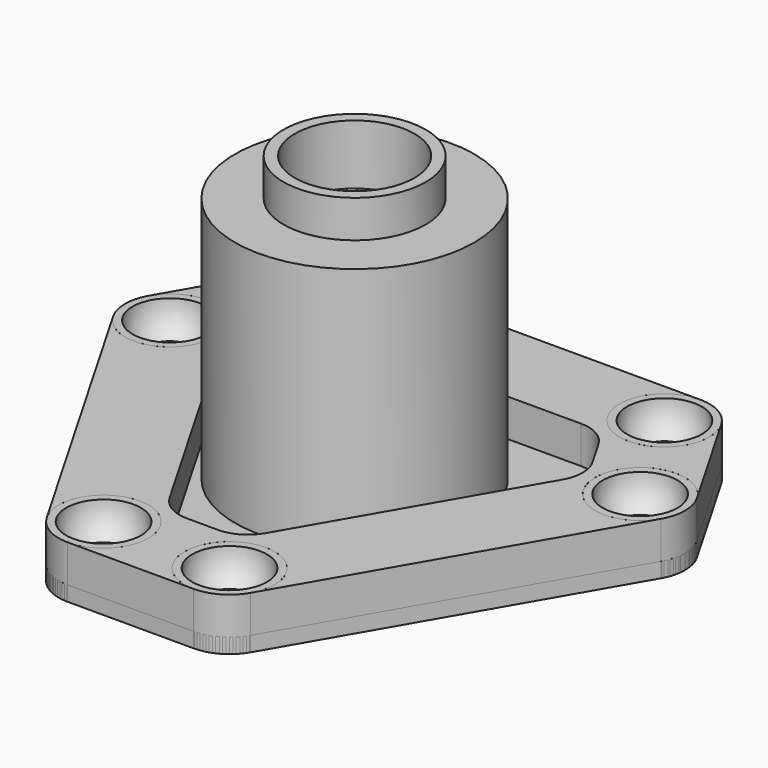
from build123d import *

# Parameters (mm, degrees)
F0_R      = 6
F1_DEPTH  = 7
F2_R      = 5
F3_DEPTH  = 5
F4_R      = 4.99999
F5_R      = 4.25
F6_DEPTH  = 3
F9_COUNT  = 3
F10_R     = 4.25
F11_DEPTH = 2
F13_DEPTH = 5
F14_R     = 13
F15_DEPTH = 2.001
F16_R     = 16
F17_DEPTH = 30
F18_R     = 13
F19_DEPTH = 30.001
F20_R     = 16
F21_DEPTH = 3
F22_R     = 8
F23_DEPTH = 3
F24_R     = 9.5
F24_R_2   = 8
F25_DEPTH = 5
F28_DEPTH = 15


# Not quite as in the source:
# - a fillet or chamfer is up to 0.001 mm smaller than in the source, because OpenCascade refuses the exact size


with BuildPart() as f1:
    # F0 (on Top) → F1 (new body)
    with BuildSketch(Plane.XY):
        with Locations((-23, 23)):
            Circle(F0_R)
    extrude(amount=F1_DEPTH)

    # F2 (on face) → F3 (cut)
    with BuildSketch(Plane.XY.offset(7)):
        with Locations((-23, 23)):
            Circle(F2_R)
    extrude(amount=-F3_DEPTH, mode=Mode.SUBTRACT)

    # F4 (radius 5 in the source; OpenCascade refuses exactly that, so slightly less here)
    f4_edges = [f1.edges().sort_by_distance(p)[0] for p in [
        (-28, 23, 2),
    ]]
    fillet(f4_edges, radius=F4_R)

    # F5 (on face) → F6 (cut)
    with BuildSketch(Plane(origin=(0, 0, 0), x_dir=(1, 0, 0), z_dir=(0, 0, -1))):
        with Locations((-23, -23)):
            Circle(F5_R)
    extrude(amount=-F6_DEPTH, mode=Mode.SUBTRACT)


with BuildPart() as f7_1:
    # F7: instance of F1
    add(f1.part.mirror(Plane.YZ))


with BuildPart() as f9_1:
    # F9: instance of F1
    add(f1.part.rotate(Axis((0, 0, 26.5737418085), (0, 0, 1)), 1 * 360 / F9_COUNT))


with BuildPart() as f9_2:
    # F9: instance of F1
    add(f1.part.rotate(Axis((0, 0, 26.5737418085), (0, 0, 1)), 2 * 360 / F9_COUNT))


with BuildPart() as f9_3:
    # F9: instance of F7_1
    add(f7_1.part.rotate(Axis((0, 0, 26.5737418085), (0, 0, 1)), 1 * 360 / F9_COUNT))


with BuildPart() as f9_4:
    # F9: instance of F7_1
    add(f7_1.part.rotate(Axis((0, 0, 26.5737418085), (0, 0, 1)), 2 * 360 / F9_COUNT))


with BuildPart() as f11:
    # F10 (on Top) → F11 (new body)
    with BuildSketch(Plane.XY):
        with BuildLine():
            ThreePointArc((29, 23), (18.7573593129, 18.7573593129), (23, 29))
            Line((23, 29), (-23, 29))
            ThreePointArc((-23, 29), (-18.7573593129, 27.2426406871), (-17, 23))
            ThreePointArc((-17, 23), (-24.5529142706, 17.2044450423), (-28.1961524227, 26))
            Line((-28.1961524227, 26), (-36.6147367097, 11.418584287))
            ThreePointArc((-36.6147367097, 11.418584287), (-29.8656700164, 14.2141392448), (-25.418584287, 8.418584287))
            ThreePointArc((-25.418584287, 8.418584287), (-29.8656700164, 2.6230293293), (-36.6147367097, 5.418584287))
            Line((-36.6147367097, 5.418584287), (-13.6147367097, -34.418584287))
            ThreePointArc((-13.6147367097, -34.418584287), (-9.9714985577, -25.6230293293), (-2.418584287, -31.418584287))
            ThreePointArc((-2.418584287, -31.418584287), (-4.1759435999, -35.6612249742), (-8.418584287, -37.418584287))
            Line((-8.418584287, -37.418584287), (8.418584287, -37.418584287))
            ThreePointArc((8.418584287, -37.418584287), (4.1759435999, -27.1759435999), (14.418584287, -31.418584287))
            ThreePointArc((14.418584287, -31.418584287), (14.2141392448, -32.9714985577), (13.6147367097, -34.418584287))
            Line((13.6147367097, -34.418584287), (36.6147367097, 5.418584287))
            ThreePointArc((36.6147367097, 5.418584287), (25.418584287, 8.418584287), (36.6147367097, 11.418584287))
            Line((36.6147367097, 11.418584287), (28.1961524227, 26))
            ThreePointArc((28.1961524227, 26), (28.7955549577, 24.5529142706), (29, 23))
        make_face()
        with BuildLine():
            ThreePointArc((28.1961524227, 26), (26, 28.1961524227), (23, 29))
            ThreePointArc((23, 29), (18.7573593129, 18.7573593129), (29, 23))
            ThreePointArc((29, 23), (28.7955549577, 24.5529142706), (28.1961524227, 26))
        make_face()
        with Locations((23, 23)):
            Circle(F10_R, mode=Mode.SUBTRACT)
        with BuildLine():
            ThreePointArc((-17, 23), (-18.7573593129, 27.2426406871), (-23, 29))
            ThreePointArc((-23, 29), (-26, 28.1961524227), (-28.1961524227, 26))
            ThreePointArc((-28.1961524227, 26), (-24.5529142706, 17.2044450423), (-17, 23))
        make_face()
        with Locations((-23, 23)):
            Circle(F10_R, mode=Mode.SUBTRACT)
        with BuildLine():
            ThreePointArc((37.418584287, 8.418584287), (37.2141392448, 9.9714985577), (36.6147367097, 11.418584287))
            ThreePointArc((36.6147367097, 11.418584287), (25.418584287, 8.418584287), (36.6147367097, 5.418584287))
            ThreePointArc((36.6147367097, 5.418584287), (37.2141392448, 6.8656700164), (37.418584287, 8.418584287))
        make_face()
        with Locations((31.418584287, 8.418584287)):
            Circle(F10_R, mode=Mode.SUBTRACT)
        with BuildLine():
            ThreePointArc((-25.418584287, 8.418584287), (-29.8656700164, 14.2141392448), (-36.6147367097, 11.418584287))
            ThreePointArc((-36.6147367097, 11.418584287), (-37.418584287, 8.418584287), (-36.6147367097, 5.418584287))
            ThreePointArc((-36.6147367097, 5.418584287), (-29.8656700164, 2.6230293293), (-25.418584287, 8.418584287))
        make_face()
        with Locations((-31.418584287, 8.418584287)):
            Circle(F10_R, mode=Mode.SUBTRACT)
        with BuildLine():
            ThreePointArc((8.418584287, -37.418584287), (11.418584287, -36.6147367097), (13.6147367097, -34.418584287))
            ThreePointArc((13.6147367097, -34.418584287), (14.2141392448, -32.9714985577), (14.418584287, -31.418584287))
            ThreePointArc((14.418584287, -31.418584287), (4.1759435999, -27.1759435999), (8.418584287, -37.418584287))
        make_face()
        with Locations((8.418584287, -31.418584287)):
            Circle(F10_R, mode=Mode.SUBTRACT)
        with BuildLine():
            ThreePointArc((-2.418584287, -31.418584287), (-9.9714985577, -25.6230293293), (-13.6147367097, -34.418584287))
            ThreePointArc((-13.6147367097, -34.418584287), (-11.418584287, -36.6147367097), (-8.418584287, -37.418584287))
            ThreePointArc((-8.418584287, -37.418584287), (-4.1759435999, -35.6612249742), (-2.418584287, -31.418584287))
        make_face()
        with Locations((-8.418584287, -31.418584287)):
            Circle(F10_R, mode=Mode.SUBTRACT)
    extrude(amount=F11_DEPTH)

    # F14 (on face) → F15 (cut, through all)
    with BuildSketch(Plane.XY.offset(2)):
        Circle(F14_R)
    extrude(amount=-F15_DEPTH, mode=Mode.SUBTRACT)

    # F16 (on face) → F17 (join)
    with BuildSketch(Plane.XY.offset(2)):
        Circle(F16_R)
    extrude(amount=F17_DEPTH)

    # F18 (on face) → F19 (cut, through all)
    with BuildSketch(Plane(origin=(0, 0, 2), x_dir=(1, 0, 0), z_dir=(0, 0, -1))):
        Circle(F18_R)
    extrude(amount=-F19_DEPTH, mode=Mode.SUBTRACT)

    # F20 (on face) → F21 (join)
    with BuildSketch(Plane.XY.offset(32)):
        Circle(F20_R)
    extrude(amount=F21_DEPTH)

    # F22 (on face) → F23 (cut)
    with BuildSketch(Plane.XY.offset(35)):
        Circle(F22_R)
    extrude(amount=-F23_DEPTH, mode=Mode.SUBTRACT)

    # F24 (on face) → F25 (join)
    with BuildSketch(Plane.XY.offset(35)):
        Circle(F24_R)
        Circle(F24_R_2, mode=Mode.SUBTRACT)
    extrude(amount=F25_DEPTH)

    # F27 (on offset) → F28 (cut)
    with BuildSketch(Plane(origin=(-15.0849364905, 8.7092921435, 0), x_dir=(0.5, 0.8660254038, 0), z_dir=(0.8660254038, -0.5, 0))):
        with BuildLine():
            Line((-1, 30), (-1, 8))
            ThreePointArc((-1, 8), (0, 7), (1, 8))
            Line((1, 8), (1, 30))
            ThreePointArc((1, 30), (0, 31), (-1, 30))
        make_face()
        with BuildLine():
            Line((4, 30), (4, 8))
            ThreePointArc((4, 8), (5, 7), (6, 8))
            Line((6, 8), (6, 30))
            ThreePointArc((6, 30), (5, 31), (4, 30))
        make_face()
        with BuildLine():
            Line((9, 30), (9, 8))
            ThreePointArc((9, 8), (10, 7), (11, 8))
            Line((11, 8), (11, 30))
            ThreePointArc((11, 30), (10, 31), (9, 30))
        make_face()
        with BuildLine():
            Line((-5.9996371421, 30.0602365921), (-5.9996371421, 8.0602365921))
            ThreePointArc((-5.9996371421, 8.0602365921), (-4.9996371421, 7.0602365921), (-3.9996371421, 8.0602365921))
            Line((-3.9996371421, 8.0602365921), (-3.9996371421, 30.0602365921))
            ThreePointArc((-3.9996371421, 30.0602365921), (-4.9996371421, 31.0602365921), (-5.9996371421, 30.0602365921))
        make_face()
        with BuildLine():
            Line((-10.9992742843, 30.1204731841), (-10.9992742843, 8.1204731841))
            ThreePointArc((-10.9992742843, 8.1204731841), (-9.9992742843, 7.1204731841), (-8.9992742843, 8.1204731841))
            Line((-8.9992742843, 8.1204731841), (-8.9992742843, 30.1204731841))
            ThreePointArc((-8.9992742843, 30.1204731841), (-9.9992742843, 31.1204731841), (-10.9992742843, 30.1204731841))
        make_face()
    extrude(amount=F28_DEPTH, mode=Mode.SUBTRACT)


with BuildPart() as f13:
    # F12 (on face) → F13 (new body)
    with BuildSketch(Plane.XY.offset(2)):
        with BuildLine():
            ThreePointArc((28.1961524227, 26), (28.7955549577, 24.5529142706), (29, 23))
            ThreePointArc((29, 23), (18.7573593129, 18.7573593129), (23, 29))
            Line((23, 29), (-23, 29))
            ThreePointArc((-23, 29), (-18.7573593129, 27.2426406871), (-17, 23))
            ThreePointArc((-17, 23), (-24.5529142706, 17.2044450423), (-28.1961524227, 26))
            Line((-28.1961524227, 26), (-36.6147367097, 11.418584287))
            ThreePointArc((-36.6147367097, 11.418584287), (-29.8656700164, 14.2141392448), (-25.418584287, 8.418584287))
            ThreePointArc((-25.418584287, 8.418584287), (-29.8656700164, 2.6230293293), (-36.6147367097, 5.418584287))
            Line((-36.6147367097, 5.418584287), (-13.6147367097, -34.418584287))
            ThreePointArc((-13.6147367097, -34.418584287), (-9.9714985577, -25.6230293293), (-2.418584287, -31.418584287))
            ThreePointArc((-2.418584287, -31.418584287), (-4.1759435999, -35.6612249742), (-8.418584287, -37.418584287))
            Line((-8.418584287, -37.418584287), (8.418584287, -37.418584287))
            ThreePointArc((8.418584287, -37.418584287), (4.1759435999, -27.1759435999), (14.418584287, -31.418584287))
            ThreePointArc((14.418584287, -31.418584287), (14.2141392448, -32.9714985577), (13.6147367097, -34.418584287))
            Line((13.6147367097, -34.418584287), (36.6147367097, 5.418584287))
            ThreePointArc((36.6147367097, 5.418584287), (25.418584287, 8.418584287), (36.6147367097, 11.418584287))
            Line((36.6147367097, 11.418584287), (28.1961524227, 26))
        make_face()
        with BuildLine():
            Line((-16.6491470389, 17), (16.6491470389, 17))
            ThreePointArc((16.6491470389, 17), (19.1491470389, 16.3301270189), (20.9792740578, 14.5))
            Line((20.9792740578, 14.5), (23.0470053838, 10.918584287))
            ThreePointArc((23.0470053838, 10.918584287), (23.7168783649, 8.418584287), (23.0470053838, 5.918584287))
            Line((23.0470053838, 5.918584287), (6.3978583449, -22.918584287))
            ThreePointArc((6.3978583449, -22.918584287), (4.567731326, -24.748711306), (2.067731326, -25.418584287))
            Line((2.067731326, -25.418584287), (-2.067731326, -25.418584287))
            ThreePointArc((-2.067731326, -25.418584287), (-4.567731326, -24.748711306), (-6.3978583449, -22.918584287))
            Line((-6.3978583449, -22.918584287), (-23.0470053838, 5.918584287))
            ThreePointArc((-23.0470053838, 5.918584287), (-23.7168783649, 8.418584287), (-23.0470053838, 10.918584287))
            Line((-23.0470053838, 10.918584287), (-20.9792740578, 14.5))
            ThreePointArc((-20.9792740578, 14.5), (-19.1491470389, 16.3301270189), (-16.6491470389, 17))
        make_face(mode=Mode.SUBTRACT)
    extrude(amount=F13_DEPTH)


solid = Compound([f1.part, f7_1.part, f9_1.part, f9_2.part, f9_3.part, f9_4.part, f11.part, f13.part])
